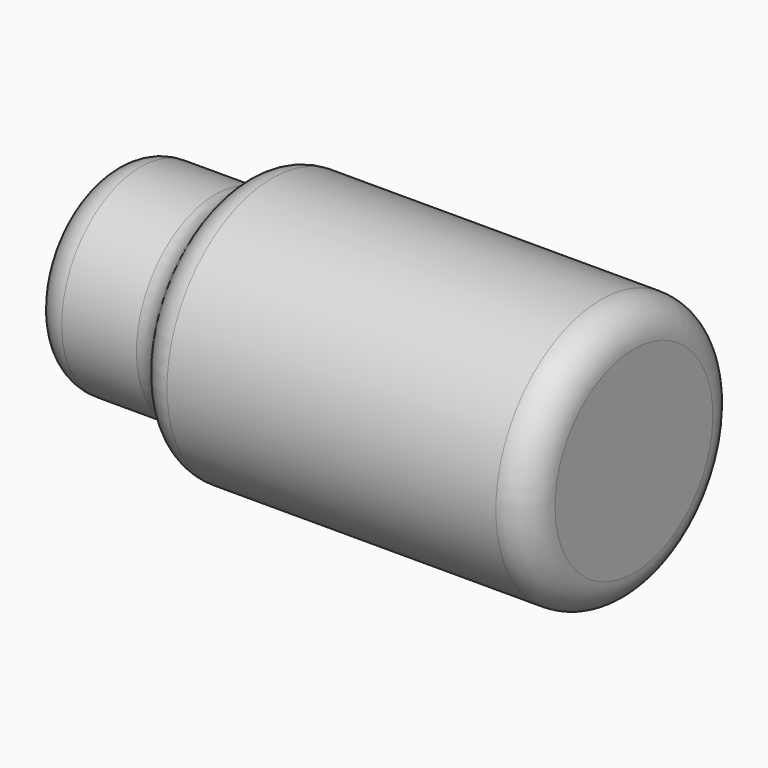
from build123d import *

# Parameters (mm, degrees)
F0_W     = 60
F0_H     = 20
F2_R     = 5
F3_DEPTH = 20
F4_R     = 5


with BuildPart() as f1:
    # F0 (on Front) → F1 (revolve)
    with BuildSketch(Plane.XZ):
        with Locations((-30, 10)):
            Rectangle(F0_W, F0_H)
    revolve(axis=Axis((-30, 0, 0), (-1, 0, 0)))

    # F2
    f2_edges = [f1.edges().sort_by_distance(p)[0] for p in [
        (-60, 0, -20),
        (0, 0, -20),
    ]]
    fillet(f2_edges, radius=F2_R)

    # F3 (add): a face of the model
    f3_faces = [f1.faces().sort_by_distance(p)[0] for p in [
        (-60, 0, 0),
    ]]
    extrude(f3_faces, amount=F3_DEPTH)

    # F4
    f4_edges = [f1.edges().sort_by_distance(p)[0] for p in [
        (-60, 0, -15),
        (-80, 0, -15),
    ]]
    fillet(f4_edges, radius=F4_R)


solid = f1.part
